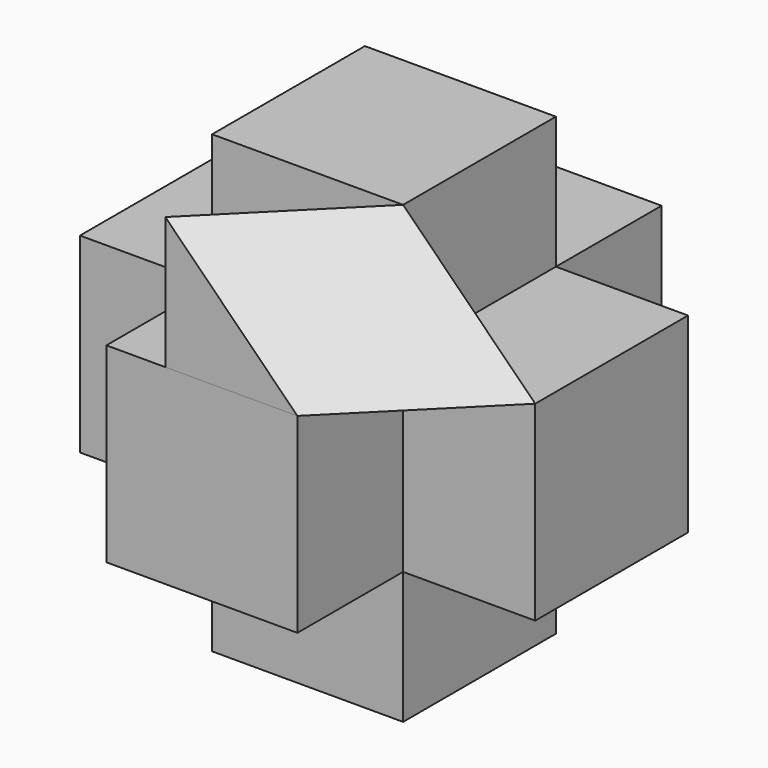
from build123d import *

# Parameters (mm, degrees)
F0_W     = 32.714
F0_H     = 32.714
F1_DEPTH = 16.357
F2_DEPTH = 22.627
F3_DEPTH = 22.627
F4_DEPTH = 22.627
F5_DEPTH = 22.627
F6_DEPTH = 22.627
F7_DEPTH = 22.627


with BuildPart() as f1:
    # F0 (on Front) → F1 (new body, symmetric)
    with BuildSketch(Plane.XZ):
        Rectangle(F0_W, F0_H)
    extrude(amount=F1_DEPTH, both=True)


with BuildPart() as f2:
    # F2 (new): a face of the model
    f2_faces = [f1.part.faces().sort_by_distance(p)[0] for p in [
        (-16.357, 0, 0),
    ]]
    extrude(f2_faces, amount=F2_DEPTH)


with BuildPart() as f3:
    # F3 (new): a face of the model
    f3_faces = [f1.part.faces().sort_by_distance(p)[0] for p in [
        (0, -16.357, 0),
    ]]
    extrude(f3_faces, amount=F3_DEPTH)


with BuildPart() as f4:
    # F4 (new): a face of the model
    f4_faces = [f1.part.faces().sort_by_distance(p)[0] for p in [
        (16.357, 0, 0),
    ]]
    extrude(f4_faces, amount=F4_DEPTH)


with BuildPart() as f5:
    # F5 (new): a face of the model
    f5_faces = [f1.part.faces().sort_by_distance(p)[0] for p in [
        (0, 16.357, 0),
    ]]
    extrude(f5_faces, amount=F5_DEPTH)


with BuildPart() as f6:
    # F6 (new): a face of the model
    f6_faces = [f1.part.faces().sort_by_distance(p)[0] for p in [
        (0, 0, 16.357),
    ]]
    extrude(f6_faces, amount=F6_DEPTH)


with BuildPart() as f1_1:
    add(f1.part)

    # F7 (add): a face of the model
    f7_faces = [f1_1.faces().sort_by_distance(p)[0] for p in [
        (0, 0, -16.357),
    ]]

    add(f2.part)  # F7 merges F2

    add(f3.part)  # F7 merges F3

    add(f4.part)  # F7 merges F4

    add(f5.part)  # F7 merges F5
    extrude(f7_faces, amount=F7_DEPTH)

    # F8: union F6
    add(f6.part)


with BuildPart() as f11:
    # F11: sweep along a path in F10
    with BuildLine(Plane.XY.offset(16.357)) as f11_path:
        Line((38.9848339741, -16.357), (16.357, -38.984))
    # F9 (on face) → F11 (sweep)
    with BuildSketch(Plane.XZ.offset(16.357)):
        Polygon((16.357, 38.984), (16.357, 16.357), (38.9846925693, 16.357), align=None)
    sweep(path=f11_path.line)


solid = Compound([f1_1.part, f11.part])
